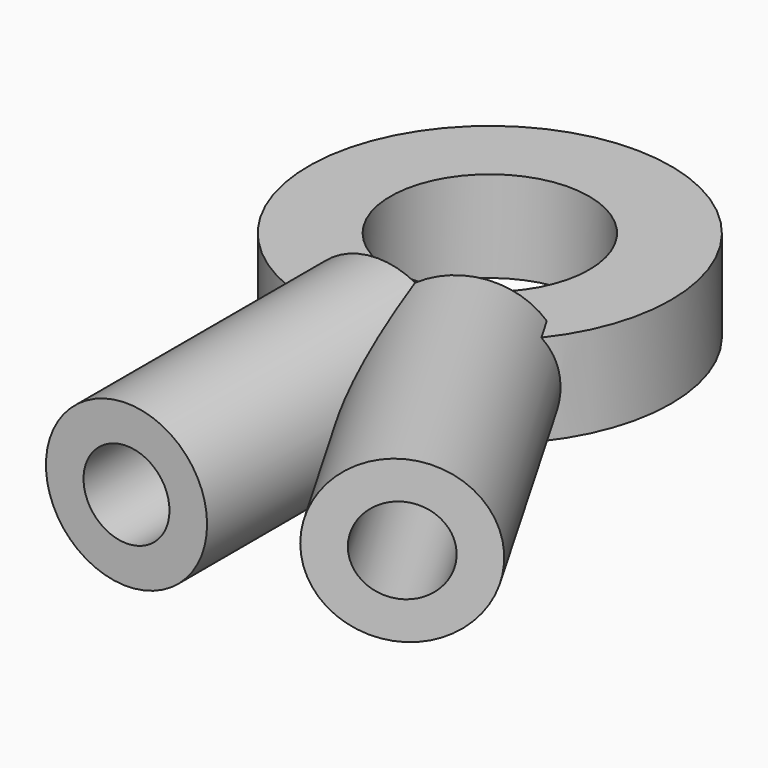
from build123d import *

# Parameters (mm, degrees)
F0_R     = 8.435
F0_R_2   = 4.625
F1_DEPTH = 2.125
F3_R     = 3.75
F3_R_2   = 2
F4_DEPTH = 14.605
F5_R     = 2
F6_DEPTH = 10.16


# Not quite as in the source:
# - a pattern or mirror of a feature is missing from the dataset's text; its kind, count and spacing are read off the source's solid


with BuildPart() as f1:
    # F0 (on Top) → F1 (new body, symmetric)
    with BuildSketch(Plane.XY):
        Circle(F0_R)
        Circle(F0_R_2, mode=Mode.SUBTRACT)
    extrude(amount=F1_DEPTH, both=True)

    # F3 (on offset) → F4 (join)
    with BuildSketch(Plane.XZ.offset(6.53)):
        Circle(F3_R)
        Circle(F3_R_2, mode=Mode.SUBTRACT)
        Circle(F3_R_2)
    f4 = extrude(amount=F4_DEPTH)

    # F4_copies: F4 across plane
    add(f4.mirror(Plane(origin=(0, 0, 0), x_dir=(-0.2588190451, 0.9659258263, 0), z_dir=(0.9659258263, 0.2588190451, 0))))

    # F5 (on face) → F6 (cut)
    with BuildSketch(Plane.XZ.offset(21.135)):
        Circle(F5_R)
    f6 = extrude(amount=-F6_DEPTH, mode=Mode.SUBTRACT)

    # F6_copies: F6 across plane
    add(f6.mirror(Plane(origin=(0, 0, 0), x_dir=(-0.2588190451, 0.9659258263, 0), z_dir=(0.9659258263, 0.2588190451, 0))), mode=Mode.SUBTRACT)


solid = f1.part
